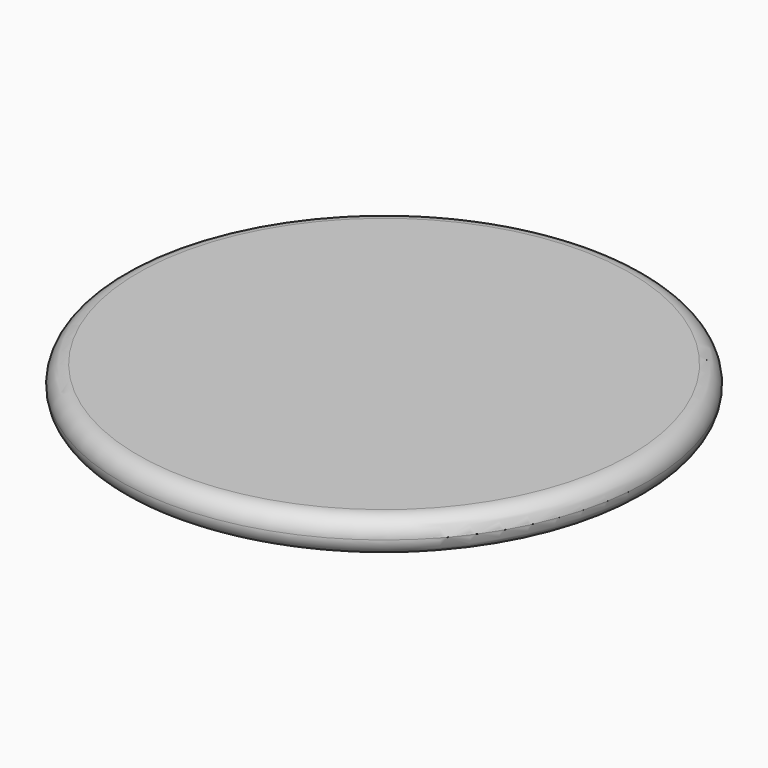
from build123d import *

# Parameters (mm, degrees)
F0_R     = 38.1
F1_DEPTH = 5.08
F2_R     = 2.53999


# Not quite as in the source:
# - a fillet or chamfer is up to 0.001 mm smaller than in the source, because OpenCascade refuses the exact size


with BuildPart() as f1:
    # F0 (on Top) → F1 (new body)
    with BuildSketch(Plane.XY):
        with Locations((-59.4195388258, 16.4489131421)):
            Circle(F0_R)
    extrude(amount=F1_DEPTH)

    # F2 (radius 2.54 in the source; OpenCascade refuses exactly that, so slightly less here)
    f2_edges = [f1.edges().sort_by_distance(p)[0] for p in [
        (-97.519539, 16.448913, 0),
        (-97.519539, 16.448913, 5.08),
    ]]
    fillet(f2_edges, radius=F2_R)


solid = f1.part
